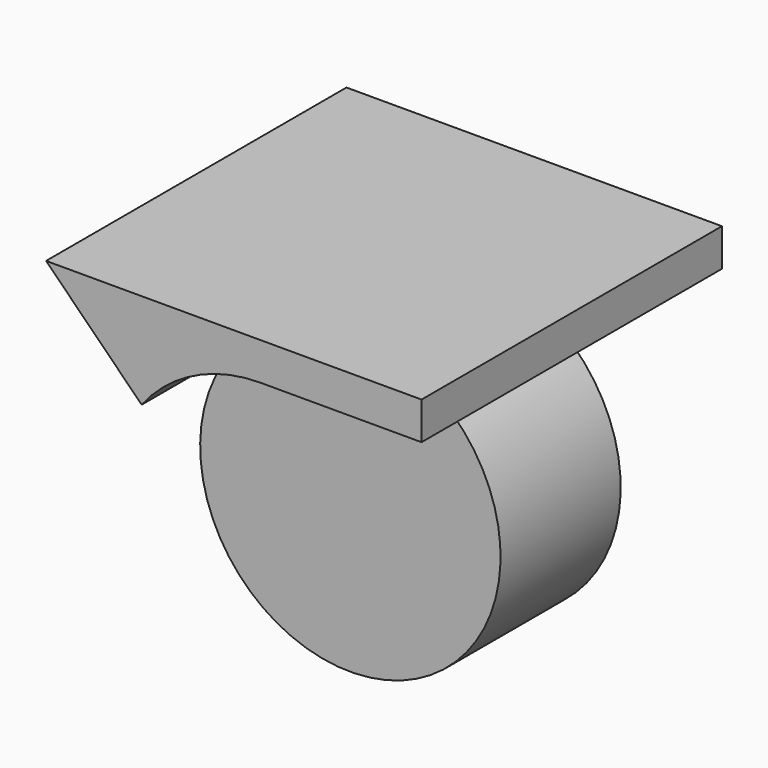
from build123d import *

# Parameters (mm, degrees)
F1_DEPTH = 40
F3_DEPTH = 30
F5_DEPTH = 30


with BuildPart() as f1:
    # F0 (on Front) → F1 (new body)
    with BuildSketch(Plane.XZ):
        with BuildLine():
            Line((-57.0404038358, 50), (-31.5845597131, 24.5441558773))
            ThreePointArc((-31.5845597131, 24.5441558773), (17.5817201222, -35.9288619016), (0, 40))
            Line((0, 40), (42.9595961642, 40))
            Line((42.9595961642, 40), (42.9595961642, 50))
            Line((42.9595961642, 50), (-57.0404038358, 50))
        make_face()
    extrude(amount=F1_DEPTH)

    # F2 (on face) → F3 (join)
    with BuildSketch(Plane.XZ.offset(40)):
        with BuildLine():
            ThreePointArc((-31.5845597131, 24.5441558773), (-17.5817201222, 35.9288619016), (0, 40))
            Line((0, 40), (42.9595961642, 40))
            Line((42.9595961642, 40), (42.9595961642, 50))
            Line((42.9595961642, 50), (-57.0404038358, 50))
            Line((-57.0404038358, 50), (-31.5845597131, 24.5441558773))
        make_face()
    extrude(amount=F3_DEPTH)

    # F4 (on face) → F5 (join)
    with BuildSketch(Plane(origin=(0, 0, 0), x_dir=(-1, 0, 0), z_dir=(0, 1, 0))):
        with BuildLine():
            ThreePointArc((0, 40), (17.5817201222, 35.9288619016), (31.5845597131, 24.5441558773))
            Line((31.5845597131, 24.5441558773), (57.0404038358, 50))
            Line((57.0404038358, 50), (-42.9595961642, 50))
            Line((-42.9595961642, 50), (-42.9595961642, 40))
            Line((-42.9595961642, 40), (0, 40))
        make_face()
    extrude(amount=F5_DEPTH)


solid = f1.part
